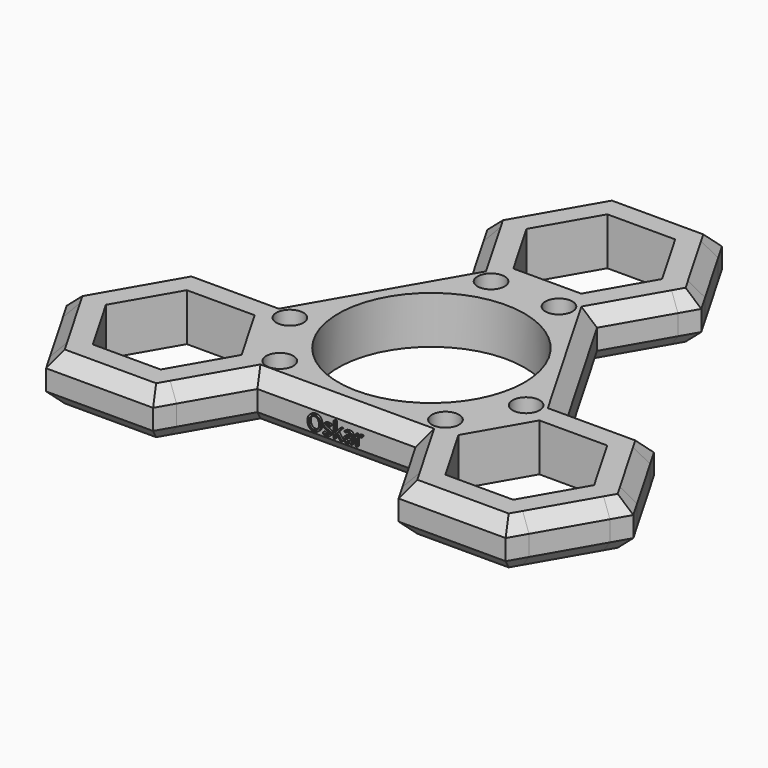
from build123d import *

# Parameters (mm, degrees)
F0_R         = 2
F0_R_2       = 13.7254526773
F1_DEPTH     = 7
F2_SIZE      = 2
F3_TEXT_SIZE = 2.990658201
F4_DEPTH     = 0.33


# Not quite as in the source:
# - Text() gives the source's letters only with a copy of the font that has no kerning and outlines rounded to 1/6400 em; it was checked with that copy


with BuildPart() as f1:
    # F0 (on Top) → F1 (new body)
    with BuildSketch(Plane.XY):
        Polygon((5, 43.6602532864), (-5, 43.6602532864), (-7.8867517548, 43.6602532864), (-9.3301517696, 41.1602111251), (-14.3300193047, 32.5001865232), (-15.7735025163, 30.0000002608), (-14.3283879783, 27.4969884581), (-9.3301267743, 18.8397461034), (-20.9807621135, -1.3397459406), (-30.9807621135, -1.3397459406), (-33.8675126262, -1.3397459406), (-35.3108885168, -3.8397463176), (-40.3108885168, -12.5000003554), (-41.754263791, -14.9999996647), (-40.3108882265, -17.4999994769), (-35.3108882265, -26.1602535148), (-33.8675119541, -28.660254553), (-30.9807621135, -28.660254553), (-20.9807621135, -28.660254553), (-18.0940115266, -28.660254553), (-16.6494248616, -26.1581570532), (-11.6506354408, -17.4999998001), (11.6506354408, -17.4999998001), (16.6504818564, -26.1599878219), (18.0940115266, -28.660254553), (20.9807621135, -28.660254553), (30.9807621135, -28.660254553), (33.8675119541, -28.660254553), (35.3108882265, -26.1602535148), (40.3092975257, -17.5027546514), (41.754263791, -14.9999996647), (40.3106246425, -12.4995433117), (35.3125127288, -3.8425595353), (33.8675126262, -1.3397459406), (30.9807621135, -1.3397459406), (20.9807621135, -1.3397459406), (9.3301267743, 18.8397461034), (14.3301234728, 27.4999944228), (15.7735025163, 30.0000002608), (14.3293581372, 32.5013316988), (9.330201807, 41.1601244578), (7.8867517548, 43.6602532864), align=None)
        Polygon((-30.9807621135, -6.3397459622), (-20.9807621135, -6.3397459622), (-15.9807621135, -15), (-20.9807621135, -23.6602540378), (-30.9807621135, -23.6602540378), (-35.9807621135, -15), align=None, mode=Mode.SUBTRACT)
        with Locations((-11.607334069, -13.4249998588)):
            Circle(F0_R, mode=Mode.SUBTRACT)
        with Locations((-17.430057958, -4.2897459622)):
            Circle(F0_R, mode=Mode.SUBTRACT)
        Circle(F0_R_2, mode=Mode.SUBTRACT)
        with Locations((12.430057958, -12.95)):
            Circle(F0_R, mode=Mode.SUBTRACT)
        Polygon((20.9807621135, -23.6602540378), (15.9807621135, -15), (20.9807621135, -6.3397459622), (30.9807621135, -6.3397459622), (35.9807621135, -15), (30.9807621135, -23.6602540378), align=None, mode=Mode.SUBTRACT)
        with Locations((17.430057958, -4.3397459622)):
            Circle(F0_R, mode=Mode.SUBTRACT)
        with Locations((-5, 17.2397459622)):
            Circle(F0_R, mode=Mode.SUBTRACT)
        Polygon((10, 30), (5, 21.3397459622), (-5, 21.3397459622), (-10, 30), (-5, 38.6602540378), (5, 38.6602540378), align=None, mode=Mode.SUBTRACT)
        with Locations((5, 17.2397459622)):
            Circle(F0_R, mode=Mode.SUBTRACT)
    extrude(amount=F1_DEPTH)

    # F2
    f2_edges = [f1.edges().sort_by_distance(p)[0] for p in [
        (-11.830127, 36.830127, 7),
        (0, 43.660253, 7),
        (-12.551815, 24.419873, 7),
        (11.830127, 36.830127, 7),
        (12.551815, 24.419873, 7),
        (15.155444, 8.75, 7),
        (27.424137, -1.339746, 7),
        (37.810888, -8.169873, 7),
        (37.810888, -21.830127, 7),
        (25.980762, -28.660255, 7),
        (14.872323, -23.080127, 7),
        (0, -17.5, 7),
        (-14.872323, -23.080127, 7),
        (-25.980762, -28.660255, 7),
        (-37.810888, -21.830127, 7),
        (-37.810888, -8.169873, 7),
        (-27.424137, -1.339746, 7),
        (-15.155444, 8.75, 7),
        (-27.424137, -1.339746, 0),
        (-37.810888, -8.169873, 0),
        (-37.810888, -21.830127, 0),
        (-25.980762, -28.660255, 0),
        (-14.872323, -23.080127, 0),
        (0, -17.5, 0),
        (14.872323, -23.080127, 0),
        (25.980762, -28.660255, 0),
        (37.810888, -21.830127, 0),
        (37.810888, -8.169873, 0),
        (27.424137, -1.339746, 0),
        (15.155444, 8.75, 0),
        (12.551815, 24.419873, 0),
        (11.830127, 36.830127, 0),
        (0, 43.660253, 0),
        (-11.830127, 36.830127, 0),
        (-12.551815, 24.419873, 0),
        (-15.155444, 8.75, 0),
    ]]
    chamfer(f2_edges, length=F2_SIZE)

    # F3 (on face) → F4 (join)
    with BuildSketch(Plane.XZ.offset(17.4999998001)):
        with Locations((-4.1944310069, 2.4674960878)):
            Text('Oskar', F3_TEXT_SIZE, font='Open Sans', text_align=(TextAlign.LEFT, TextAlign.BOTTOM))
    extrude(amount=F4_DEPTH)


solid = f1.part
